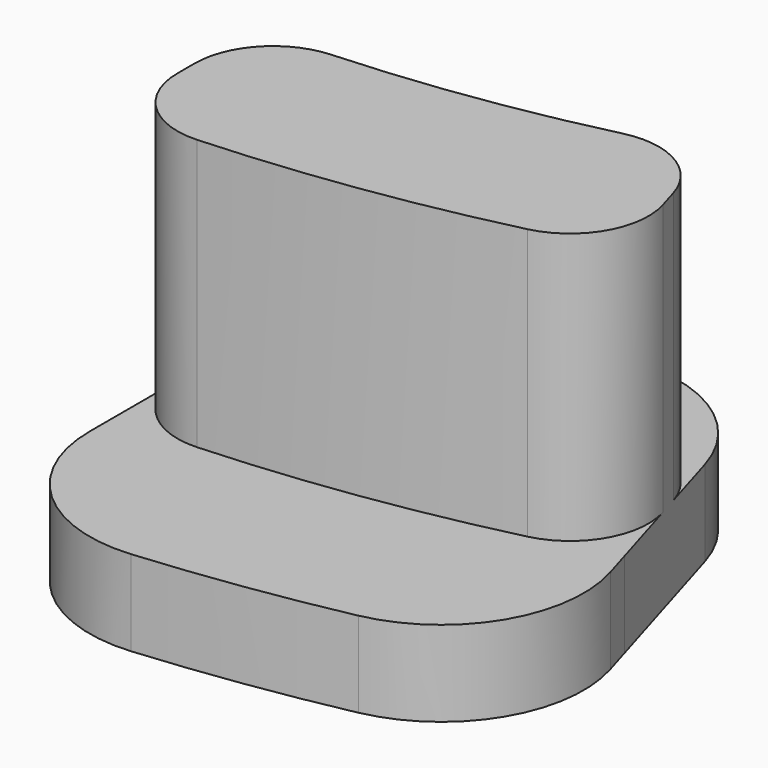
from build123d import *

# Parameters (mm, degrees)
F1_DEPTH    = 12
F2_DEPTH    = 50
F3_T1_DEPTH = 120.7987304743
F3_T3_DEPTH = 107.0496265693
F4_T1_DEPTH = 64.7830881456
F4_T3_DEPTH = 66.9231117077


# Not quite as in the source:
# - a fillet or chamfer that OpenCascade refuses, or shapes differently, is made with other operations: its cross-section is extruded or revolved along the edge and cut away or added


with BuildPart() as f1:
    # F0 (on Top) → F1 (new body)
    with BuildSketch(Plane.XY):
        with BuildLine():
            ThreePointArc((64.2798563582, -215.6225870974), (32.480131643, -222.643304522), (0, -225))
            Line((0, -225), (0, -250))
            ThreePointArc((0, -250), (36.0890351588, -247.3814494688), (71.4220626202, -239.5806523304))
            Line((71.4220626202, -239.5806523304), (64.2798563582, -215.6225870974))
        make_face()
        with BuildLine():
            ThreePointArc((57.1376500962, -191.6645218643), (28.8712281271, -197.9051595751), (0, -200))
            Line((0, -200), (0, -225))
            ThreePointArc((0, -225), (32.480131643, -222.643304522), (64.2798563582, -215.6225870974))
            Line((64.2798563582, -215.6225870974), (57.1376500962, -191.6645218643))
        make_face()
        with BuildLine():
            ThreePointArc((52.1381057128, -174.8938762012), (26.344995666, -180.5884581123), (0, -182.5))
            Line((0, -182.5), (0, -200))
            ThreePointArc((0, -200), (28.8712281271, -197.9051595751), (57.1376500962, -191.6645218643))
            Line((57.1376500962, -191.6645218643), (52.1381057128, -174.8938762012))
        make_face()
    extrude(amount=F1_DEPTH)

    # F0 (on Top) → F2 (join)
    with BuildSketch(Plane.XY):
        with BuildLine():
            ThreePointArc((57.1376500962, -191.6645218643), (28.8712281271, -197.9051595751), (0, -200))
            Line((0, -200), (0, -225))
            ThreePointArc((0, -225), (32.480131643, -222.643304522), (64.2798563582, -215.6225870974))
            Line((64.2798563582, -215.6225870974), (57.1376500962, -191.6645218643))
        make_face()
    extrude(amount=F2_DEPTH)

    # F3: fillet of radius 20 on 4 edges, made by hand

    # F3_s2 → F3_t1 (cut)
    with BuildSketch(Plane.XY.offset(-54.3993652372)):
        with BuildLine():
            ThreePointArc((21.7391304348, -249.0530268998), (6.4867215062, -243.8729803633), (0, -229.1287847478))
            Line((0, -229.1287847478), (0, -250))
            ThreePointArc((0, -250), (10.8798730474, -249.7631445239), (21.7391304348, -249.0530268998))
        make_face()
        with BuildLine():
            ThreePointArc((50.3184233293, -244.883760739), (63.4552732198, -235.5621710033), (65.4594016494, -219.5792948702))
            Line((65.4594016494, -219.5792948702), (71.4220626202, -239.5806523304))
            ThreePointArc((71.4220626202, -239.5806523304), (60.9279674657, -242.4619202689), (50.3184233293, -244.883760739))
        make_face()
    extrude(amount=F3_T1_DEPTH, mode=Mode.SUBTRACT)

    # F3_s4 → F3_t3 (cut)
    with BuildSketch(Plane.XY.offset(-47.5248132847)):
        with BuildLine():
            ThreePointArc((18.024691358, -181.6077104681), (5.1759288176, -188.0843186765), (0, -201.5099253139))
            Line((0, -201.5099253139), (0, -182.5))
            ThreePointArc((0, -182.5), (9.0233818378, -182.2767911178), (18.024691358, -181.6077104681))
        make_face()
        with BuildLine():
            ThreePointArc((34.609719823, -179.1882175082), (48.7732703354, -181.7241570951), (57.5690180175, -193.111517431))
            Line((57.5690180175, -193.111517431), (52.1381057128, -174.8938762012))
            ThreePointArc((52.1381057128, -174.8938762012), (43.42702673, -177.2578442535), (34.609719823, -179.1882175082))
        make_face()
    extrude(amount=F3_T3_DEPTH, mode=Mode.SUBTRACT)

    # F4: fillet of radius 11 on 4 edges, made by hand

    # F4_s2 → F4_t1 (cut)
    with BuildSketch(Plane.XY.offset(12)):
        with BuildLine():
            ThreePointArc((0, -210.7130750571), (3.0216525247, -203.140362758), (10.4265402844, -199.7280332294))
            Line((10.4265402844, -199.7280332294), (10.3691943128, -198.6295290467))
            ThreePointArc((10.3691943128, -198.6295290467), (5.2147333965, -198.83162866), (0.0567649923, -198.8999918998))
            Line((0.0567649923, -198.8999918998), (-1.0397817327, -199.9169455148))
            ThreePointArc((-1.0397817327, -199.9169455148), (-1.1, -201.5099253139), (-1.1, -210.7130750571))
            Line((-1.1, -210.7130750571), (0, -210.7130750571))
        make_face()
        with BuildLine():
            ThreePointArc((60.1982497665, -201.9311039069), (55.1390969064, -195.5372531202), (47.0679630938, -194.3826300115))
            Line((47.0679630938, -194.3826300115), (46.8090892968, -193.3135255465))
            ThreePointArc((46.8090892968, -193.3135255465), (51.8064632167, -192.0346332539), (56.768991531, -190.6265763228))
            Line((56.768991531, -190.6265763228), (58.1103687488, -191.2878754492))
            ThreePointArc((58.1103687488, -191.2878754492), (58.6231728877, -192.7972603555), (61.2524046367, -201.6168468313))
            Line((61.2524046367, -201.6168468313), (60.1982497665, -201.9311039069))
        make_face()
    extrude(amount=F4_T1_DEPTH, mode=Mode.SUBTRACT)

    # F4_s4 → F4_t3 (cut)
    with BuildSketch(Plane.XY.offset(12)):
        with BuildLine():
            ThreePointArc((0, -213.7171027316), (3.4243688767, -221.6926787663), (11.5654205607, -224.7025612833))
            ThreePointArc((11.5654205607, -224.7025612833), (5.7846223415, -224.9256280293), (0, -225))
            Line((0, -225), (0, -213.7171027316))
        make_face()
        with BuildLine():
            ThreePointArc((61.0564651772, -204.8099315465), (60.0533434239, -213.4314083362), (53.1114776019, -218.6416496163))
            ThreePointArc((53.1114776019, -218.6416496163), (58.7150747837, -217.2039133928), (64.2798563582, -215.6225870974))
            Line((64.2798563582, -215.6225870974), (61.0564651772, -204.8099315465))
        make_face()
    extrude(amount=F4_T3_DEPTH, mode=Mode.SUBTRACT)


solid = f1.part
